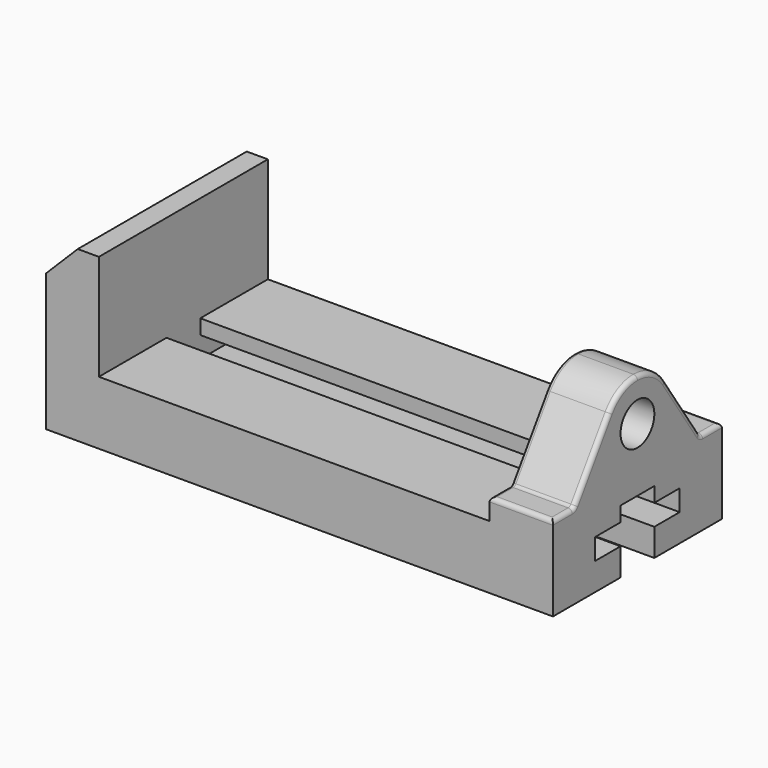
from build123d import *

# Parameters (mm, degrees)
F0_W     = 127
F0_H     = 101.6
F1_DEPTH = 304.8
F2_W     = 234.95
F2_H     = 63.5
F3_DEPTH = 127.001
F4_R     = 12.7
F5_DEPTH = 273.05
F6_SIZE  = 19.05
F7_F1_R  = 2.54
F7_F2_R  = 2.54


with BuildPart() as f1:
    # F0 (on Right) → F1 (new body)
    with BuildSketch(Plane.YZ):
        with Locations((63.5, 50.8)):
            Rectangle(F0_W, F0_H)
    extrude(amount=-F1_DEPTH)

    # F2 (on face) → F3 (cut, through all)
    with BuildSketch(Plane.XZ):
        with Locations((-155.575, 69.85)):
            Rectangle(F2_W, F2_H)
    extrude(amount=-F3_DEPTH, mode=Mode.SUBTRACT)

    # F4 (on face) → F5 (cut, through all)
    with BuildSketch(Plane.YZ):
        with Locations((63.5, 76.2)):
            Circle(F4_R)
        Polygon((50.8, 16.51), (50.8, 0), (76.2, 0), (76.2, 16.51), (95.25, 16.51), (95.25, 29.21), (76.2, 29.21), (76.2, 38.1), (50.8, 38.1), (50.8, 29.21), (31.75, 29.21), (31.75, 16.51), align=None)
        with BuildLine():
            Line((0, 101.6), (0, 50.8))
            Line((0, 50.8), (15.875, 50.8))
            Line((15.875, 50.8), (42.4065743945, 90.3501730104))
            ThreePointArc((42.4065743945, 90.3501730104), (51.5470588235, 98.6117647059), (63.5, 101.6))
            Line((63.5, 101.6), (0, 101.6))
        make_face()
        with BuildLine():
            Line((127, 101.6), (63.5, 101.6))
            ThreePointArc((63.5, 101.6), (75.4529411765, 98.6117647059), (84.5934256055, 90.3501730104))
            Line((84.5934256055, 90.3501730104), (111.125, 50.8))
            Line((111.125, 50.8), (127, 50.8))
            Line((127, 50.8), (127, 101.6))
        make_face()
    extrude(amount=-F5_DEPTH, mode=Mode.SUBTRACT)

    # F6
    f6_edges = [f1.edges().sort_by_distance(p)[0] for p in [
        (-304.8, 63.5, 101.6),
    ]]
    chamfer(f6_edges, length=F6_SIZE)

    # F7: fillet of radius 2.54 on 6 edges, made by hand

    # F7_f1
    f7_f1_edges = [f1.edges().sort_by_distance(p)[0] for p in [
        (-19.05, 15.875, 50.8),
        (-19.05, 111.125, 50.8),
    ]]
    fillet(f7_f1_edges, radius=F7_F1_R)

    # F7_f2
    f7_f2_edges = [f1.edges().sort_by_distance(p)[0] for p in [
        (0, 29.5181251442, 71.1375778547),
        (-38.1, 29.5181251442, 71.1375778547),
        (-19.05, 127, 50.8),
        (-19.05, 0, 50.8),
        (-38.1, 63.5, 101.6),
        (-38.1, 97.4818748558, 71.1375778547),
        (0, 63.5, 101.6),
        (0, 97.4818748558, 71.1375778547),
        (0, 111.284372549, 51.0988235294),
        (-38.1, 111.284372549, 51.0988235294),
        (-38.1, 15.715627451, 51.0988235294),
        (0, 15.715627451, 51.0988235294),
    ]]
    fillet(f7_f2_edges, radius=F7_F2_R)


solid = f1.part
